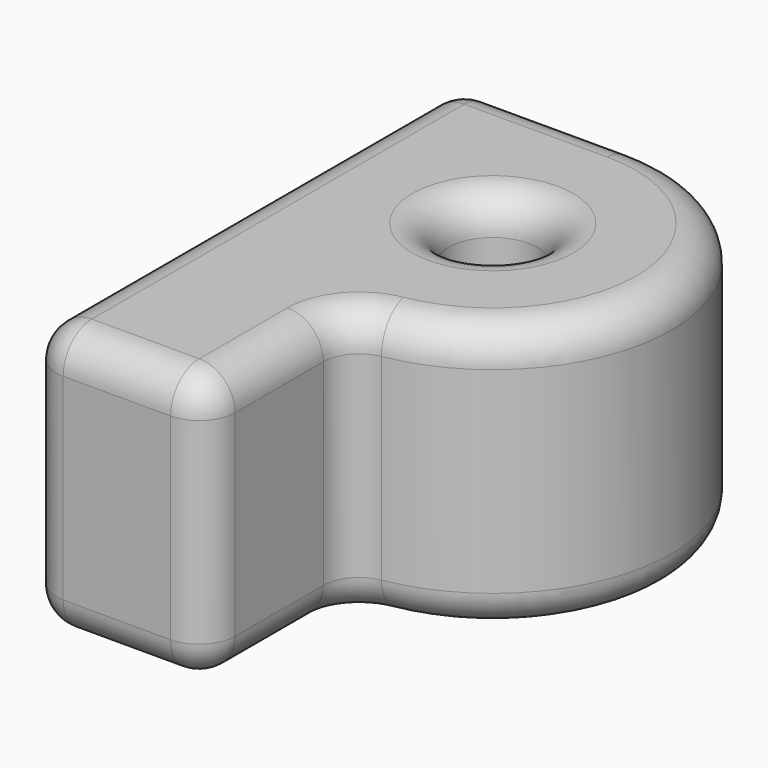
from build123d import *

# Parameters (mm, degrees)
F0_R     = 2.5
F1_DEPTH = 15
F2_R     = 2


with BuildPart() as f1:
    # F0 (on Top) → F1 (new body)
    with BuildSketch(Plane.XY):
        with BuildLine():
            Line((0, 30), (0, 0))
            Line((0, 0), (10, 0))
            Line((10, 0), (10, 10))
            ThreePointArc((10, 10), (20, 20), (10, 30))
            Line((10, 30), (0, 30))
        make_face()
        with Locations((10, 20)):
            Circle(F0_R, mode=Mode.SUBTRACT)
    extrude(amount=F1_DEPTH)

    # F2
    f2_edges = [f1.edges().sort_by_distance(p)[0] for p in [
        (5, 0, 15),
        (10, 5, 15),
        (20, 20, 15),
        (0, 15, 15),
        (0, 15, 0),
        (10, 10, 7.5),
        (10, 30, 7.5),
        (20, 20, 0),
        (7.5, 20, 0),
        (5, 0, 0),
        (0, 0, 7.5),
        (10, 0, 7.5),
        (0, 30, 7.5),
        (12.5, 20, 7.5),
        (7.5, 20, 15),
        (5, 30, 15),
        (5, 30, 0),
        (10, 5, 0),
    ]]
    fillet(f2_edges, radius=F2_R)


solid = f1.part
